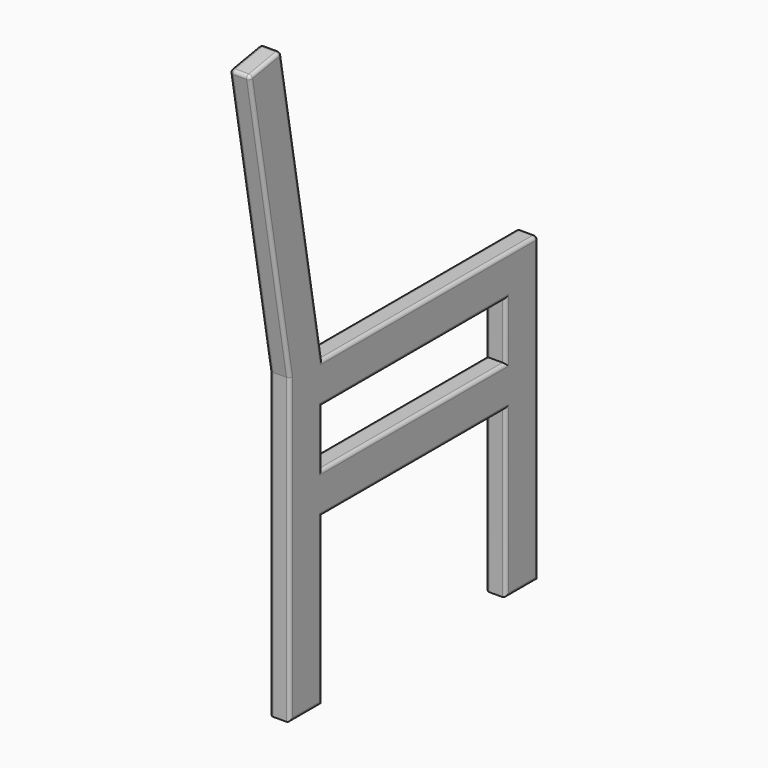
from build123d import *

# Parameters (mm, degrees)
F0_W         = 340.9255967131
F0_H         = 60
F1_DEPTH     = 30
F2_R         = 5
F3_T1_DEPTH  = 20
F3_S5_W      = 5
F3_S5_H      = 5
F3_T6_DEPTH  = 5
F3_S11_W     = 5
F3_S11_H     = 5
F3_T12_DEPTH = 5
F3_S17_W     = 5
F3_S17_H     = 5
F3_T18_DEPTH = 5
F3_S23_W     = 5
F3_S23_H     = 5
F3_T24_DEPTH = 5
F3_S29_W     = 5
F3_S29_H     = 5
F3_T30_DEPTH = 5
F3_S35_W     = 5
F3_S35_H     = 5
F3_T36_DEPTH = 5


# Not quite as in the source:
# - a fillet or chamfer that OpenCascade refuses, or shapes differently, is made with other operations: its cross-section is extruded or revolved along the edge and cut away or added


with BuildPart() as f1:
    # F0 (on Right) → F1 (new body)
    with BuildSketch(Plane.YZ):
        Polygon((-254.4838840649, 268.3866892413), (-254.4838840649, -181.6133107587), (-194.4838840649, -181.6133107587), (-194.4838840649, 64.7750496864), (-194.4838840649, 124.7750496864), (-194.4838840649, 208.3866892413), (146.4417126483, 208.3866892413), (146.4417126483, 124.7750496864), (146.4417126483, 64.7750496864), (146.4417126483, -181.6133107587), (206.4417126483, -181.6133107587), (206.4417126483, 268.3866892413), (-193.5582873517, 268.3866892413), (-270.1950266739, 703.015235674), (-329.2834918547, 692.596345014), align=None)
        with Locations((-24.0210857083, 94.7750496864)):
            Rectangle(F0_W, F0_H)
    extrude(amount=F1_DEPTH)

    # F2
    f2_edges = [f1.edges().sort_by_distance(p)[0] for p in [
        (30, -254.483884, 43.386689),
        (30, -224.483884, -181.613311),
        (30, -194.483884, -58.419131),
        (30, -24.021086, 64.77505),
        (30, 146.441713, -58.419131),
        (30, 176.441713, -181.613311),
        (30, 206.441713, 43.386689),
        (30, 6.441713, 268.386689),
        (30, -231.876657, 485.700962),
        (30, -299.739259, 697.80579),
        (30, -291.883688, 480.491517),
        (30, -194.483884, 166.580869),
        (30, -24.021086, 208.386689),
        (30, 146.441713, 166.580869),
        (30, -24.021086, 124.77505),
        (0, -254.483884, 43.386689),
        (0, -224.483884, -181.613311),
        (0, -194.483884, -58.419131),
        (0, -24.021086, 64.77505),
        (0, 146.441713, -58.419131),
        (0, 176.441713, -181.613311),
        (0, 206.441713, 43.386689),
        (0, 6.441713, 268.386689),
        (0, -231.876657, 485.700962),
        (0, -299.739259, 697.80579),
        (0, -291.883688, 480.491517),
        (0, -194.483884, 166.580869),
        (0, -24.021086, 208.386689),
        (0, 146.441713, 166.580869),
        (0, -24.021086, 124.77505),
    ]]
    fillet(f2_edges, radius=F2_R)

    # F3: fillet of radius 5 on 3 edges, made by hand

    # F3_s2 → F3_t1 (cut)
    with BuildSketch(Plane.YZ.offset(5)):
        with BuildLine():
            ThreePointArc((201.4417126483, 268.3866892413), (204.9772465542, 266.9222231472), (206.4417126483, 263.3866892413))
            Line((206.4417126483, 263.3866892413), (206.4417126483, 268.3866892413))
            Line((206.4417126483, 268.3866892413), (201.4417126483, 268.3866892413))
        make_face()
        with BuildLine():
            ThreePointArc((-275.119065439, 702.1469947856), (-271.3829423689, 701.318716242), (-269.3267857856, 698.0911969089))
            Line((-269.3267857856, 698.0911969089), (-270.1950266739, 703.015235674))
            Line((-270.1950266739, 703.015235674), (-275.119065439, 702.1469947856))
        make_face()
        with BuildLine():
            ThreePointArc((-328.4152509663, 687.6723062489), (-327.5869724227, 691.408429319), (-324.3594530896, 693.4645859023))
            Line((-324.3594530896, 693.4645859023), (-329.2834918547, 692.596345014))
            Line((-329.2834918547, 692.596345014), (-328.4152509663, 687.6723062489))
        make_face()
    extrude(amount=F3_T1_DEPTH, mode=Mode.SUBTRACT)


with BuildPart() as f3_tool4:
    # F3_s5 → F3_t6 (new body)
    with BuildSketch(Plane(origin=(0, -195.9893902892, -34.5582174406), x_dir=(1, 0, 0), z_dir=(0, -0.984807753, -0.1736481777))):
        with Locations((2.5, 736.753728574)):
            Rectangle(F3_S5_W, F3_S5_H)
    extrude(amount=F3_T6_DEPTH)

    # F3_s7 → F3_t8 (revolve, cut)
    with BuildSketch(Plane(origin=(5, -323.4912122013, 688.5405471372), x_dir=(0.7071067812, 0.122787804, -0.6963642403), z_dir=(-0.7071067812, 0.122787804, -0.6963642403))):
        with BuildLine():
            ThreePointArc((0, -5), (5, 0), (0, 5))
            Line((0, 5), (0, -5))
        make_face()
    revolve(axis=Axis((5, -323.4912122013, 688.5405471372), (0, -0.984807753, -0.1736481777)), mode=Mode.SUBTRACT)


with BuildPart() as f1_1:
    add(f1.part)

    # F3_t3: cut F3_tool4
    add(f3_tool4.part, mode=Mode.SUBTRACT)


with BuildPart() as f3_tool10:
    # F3_s11 → F3_t12 (new body)
    with BuildSketch(Plane(origin=(0, -195.9893902892, -34.5582174406), x_dir=(1, 0, 0), z_dir=(0, -0.984807753, -0.1736481777))):
        with Locations((27.5, 736.753728574)):
            Rectangle(F3_S11_W, F3_S11_H)
    extrude(amount=F3_T12_DEPTH)

    # F3_s13 → F3_t14 (revolve, cut)
    with BuildSketch(Plane(origin=(25, -323.4912122013, 688.5405471372), x_dir=(-0.7071067812, 0.122787804, -0.6963642403), z_dir=(-0.7071067812, -0.122787804, 0.6963642403))):
        with BuildLine():
            ThreePointArc((0, -5), (5, 0), (0, 5))
            Line((0, 5), (0, -5))
        make_face()
    revolve(axis=Axis((25, -323.4912122013, 688.5405471372), (0, -0.984807753, -0.1736481777)), mode=Mode.SUBTRACT)


with BuildPart() as f1_2:
    add(f1_1.part)

    # F3_t9: cut F3_tool10
    add(f3_tool10.part, mode=Mode.SUBTRACT)


with BuildPart() as f3_tool16:
    # F3_s17 → F3_t18 (new body)
    with BuildSketch(Plane(origin=(0, -127.501821912, 723.0987645778), x_dir=(1, 0, 0), z_dir=(0, -0.1736481777, 0.984807753))):
        with Locations((2.5, -146.5128425469)):
            Rectangle(F3_S17_W, F3_S17_H)
    extrude(amount=F3_T18_DEPTH)

    # F3_s19 → F3_t20 (revolve, cut)
    with BuildSketch(Plane(origin=(5, -274.2508245507, 697.2229560206), x_dir=(0.7071067812, -0.6963642403, -0.122787804), z_dir=(-0.7071067812, -0.6963642403, -0.122787804))):
        with BuildLine():
            ThreePointArc((0, -5), (5, 0), (0, 5))
            Line((0, 5), (0, -5))
        make_face()
    revolve(axis=Axis((5, -274.2508245507, 697.2229560206), (0, -0.1736481777, 0.984807753)), mode=Mode.SUBTRACT)


with BuildPart() as f1_3:
    add(f1_2.part)

    # F3_t15: cut F3_tool16
    add(f3_tool16.part, mode=Mode.SUBTRACT)


with BuildPart() as f3_tool22:
    # F3_s23 → F3_t24 (new body)
    with BuildSketch(Plane(origin=(0, -127.501821912, 723.0987645778), x_dir=(1, 0, 0), z_dir=(0, -0.1736481777, 0.984807753))):
        with Locations((27.5, -146.5128425469)):
            Rectangle(F3_S23_W, F3_S23_H)
    extrude(amount=F3_T24_DEPTH)

    # F3_s25 → F3_t26 (revolve, cut)
    with BuildSketch(Plane(origin=(25, -274.2508245507, 697.2229560206), x_dir=(-0.7071067812, -0.6963642403, -0.122787804), z_dir=(-0.7071067812, 0.6963642403, 0.122787804))):
        with BuildLine():
            ThreePointArc((0, -5), (5, 0), (0, 5))
            Line((0, 5), (0, -5))
        make_face()
    revolve(axis=Axis((25, -274.2508245507, 697.2229560206), (0, -0.1736481777, 0.984807753)), mode=Mode.SUBTRACT)


with BuildPart() as f1_4:
    add(f1_3.part)

    # F3_t21: cut F3_tool22
    add(f3_tool22.part, mode=Mode.SUBTRACT)


with BuildPart() as f3_tool28:
    # F3_s29 → F3_t30 (new body)
    with BuildSketch(Plane.XY.offset(263.3866892413)):
        with Locations((2.5, 203.9417126483)):
            Rectangle(F3_S29_W, F3_S29_H)
    extrude(amount=F3_T30_DEPTH)

    # F3_s31 → F3_t32 (revolve, cut)
    with BuildSketch(Plane(origin=(5, 201.4417126483, 263.3866892413), x_dir=(0.7071067812, -0.7071067812, 0), z_dir=(-0.7071067812, -0.7071067812, 0))):
        with BuildLine():
            ThreePointArc((0, -5), (5, 0), (0, 5))
            Line((0, 5), (0, -5))
        make_face()
    revolve(axis=Axis((5, 201.4417126483, 263.3866892413), (0, 0, 1)), mode=Mode.SUBTRACT)


with BuildPart() as f1_5:
    add(f1_4.part)

    # F3_t27: cut F3_tool28
    add(f3_tool28.part, mode=Mode.SUBTRACT)


with BuildPart() as f3_tool34:
    # F3_s35 → F3_t36 (new body)
    with BuildSketch(Plane.XY.offset(263.3866892413)):
        with Locations((27.5, 203.9417126483)):
            Rectangle(F3_S35_W, F3_S35_H)
    extrude(amount=F3_T36_DEPTH)

    # F3_s37 → F3_t38 (revolve, cut)
    with BuildSketch(Plane(origin=(25, 201.4417126483, 263.3866892413), x_dir=(-0.7071067812, -0.7071067812, 0), z_dir=(-0.7071067812, 0.7071067812, 0))):
        with BuildLine():
            ThreePointArc((0, -5), (5, 0), (0, 5))
            Line((0, 5), (0, -5))
        make_face()
    revolve(axis=Axis((25, 201.4417126483, 263.3866892413), (0, 0, 1)), mode=Mode.SUBTRACT)


with BuildPart() as f1_6:
    add(f1_5.part)

    # F3_t33: cut F3_tool34
    add(f3_tool34.part, mode=Mode.SUBTRACT)


solid = f1_6.part
